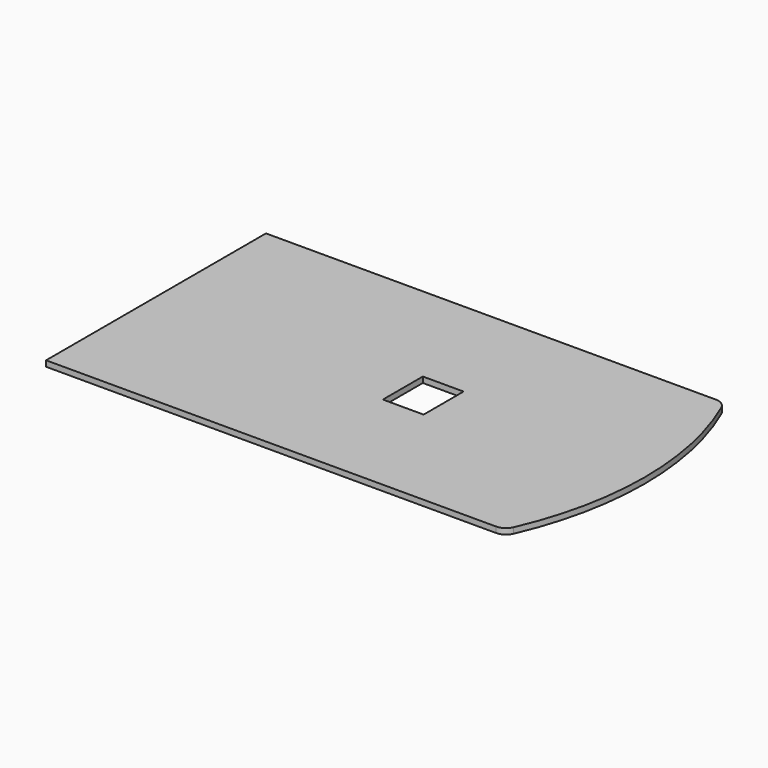
from build123d import *

# Parameters (mm, degrees)
F1_DEPTH = 28.575


# Not quite as in the source:
# - a feature names something its author has since deleted; it is built from what else it names


with BuildPart() as f1:
    # F0 (on Top) → F1 (new body)
    with BuildSketch(Plane.XY):
        with BuildLine():
            Line((1102.0184274855, 685.8), (-1143, 685.8))
            Line((-1143, 685.8), (-1143, 0))
            Line((-1143, 0), (88.9, 0))
            Line((88.9, 0), (88.9, 124.587))
            Line((88.9, 124.587), (292.1, 124.587))
            Line((292.1, 124.587), (292.1, 0))
            Line((292.1, 0), (1143, 0))
            Line((1143, 0), (1295.4, 0))
            ThreePointArc((1295.4, 0), (1261.244047213, 330.8283905438), (1160.2171388114, 647.7))
            ThreePointArc((1160.2171388114, 647.7), (1136.7988098871, 675.4279116849), (1102.0184274855, 685.8))
        make_face()
        with BuildLine():
            Line((88.9, 0), (-1143, 0))
            Line((-1143, 0), (-1143, -685.8))
            Line((-1143, -685.8), (1102.0184274855, -685.8))
            ThreePointArc((1102.0184274855, -685.8), (1136.7988098871, -675.4279116849), (1160.2171388114, -647.7))
            ThreePointArc((1160.2171388114, -647.7), (1261.244047213, -330.8283905438), (1295.4, 0))
            Line((1295.4, 0), (1143, 0))
            Line((1143, 0), (292.1, 0))
            Line((292.1, 0), (292.1, -124.587))
            Line((292.1, -124.587), (88.9, -124.587))
            Line((88.9, -124.587), (88.9, 0))
        make_face()
    extrude(amount=F1_DEPTH)


solid = f1.part
